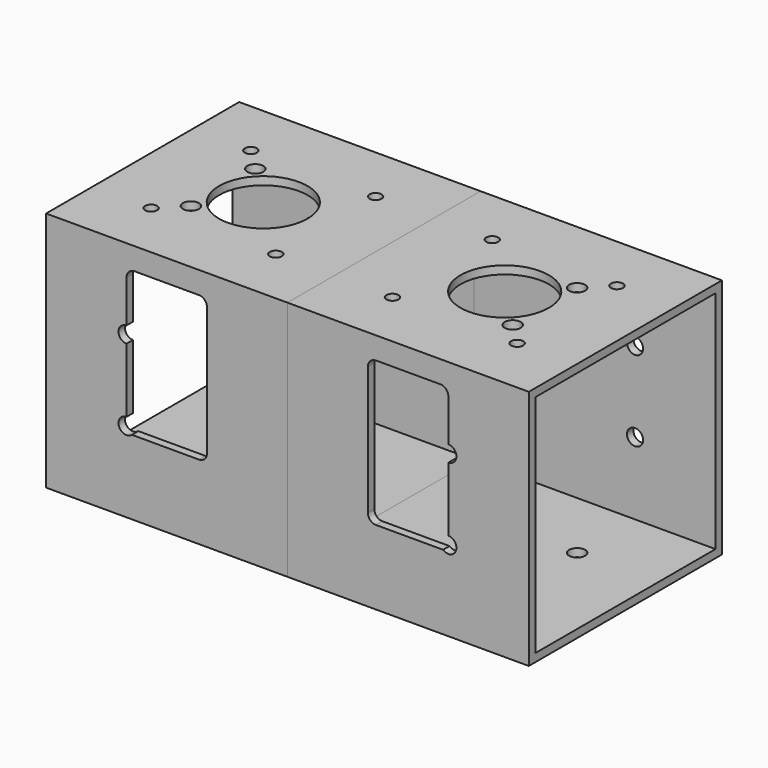
from build123d import *

# Parameters (mm, degrees)
F0_W     = 60
F0_H     = 60
F1_DEPTH = 60
F2_T     = -2
F4_D     = 4
F5_D     = 22
F5_DEPTH = 2
F5_TIP   = 6.6094668093
F6_D     = 3
F6_DEPTH = 2
F6_TIP   = 0.9012909285
F8_D     = 4
F7_W     = 20
F7_H     = 36
F9_DEPTH = 2
F10_R    = 2


with BuildPart() as f1:
    # F0 (on Right) → F1 (new body)
    with BuildSketch(Plane.YZ):
        Rectangle(F0_W, F0_H)
    extrude(amount=-F1_DEPTH)

    # F2
    f2_openings = [f1.faces().sort_by_distance(p)[0] for p in [
        (-60, 0, 0),
        (0, 0, 0),
    ]]
    offset(amount=F2_T, openings=f2_openings)

    # F4 (through all)
    with Locations(Plane.XY.offset(30)):
        with Locations((-40, 10), (-40, -10)):
            Hole(F4_D / 2)

    # F5
    with Locations(Plane.XY.offset(30)):
        with Locations((-30, 0)):
            Hole(F5_D / 2, depth=F5_DEPTH)
            with Locations((0, 0, -(F5_DEPTH + F5_TIP / 2))):  # 118° drill point
                Cone(0, F5_D / 2, F5_TIP, mode=Mode.SUBTRACT)

    # F6
    with Locations(Plane.XY.offset(30)):
        with Locations((-45.5, 15.5), (-14.5, 15.5), (-14.5, -15.5), (-45.5, -15.5)):
            Hole(F6_D / 2, depth=F6_DEPTH)
            with Locations((0, 0, -(F6_DEPTH + F6_TIP / 2))):  # 118° drill point
                Cone(0, F6_D / 2, F6_TIP, mode=Mode.SUBTRACT)

    # F8 (through all)
    with Locations(Plane.XZ.offset(30)):
        with Locations((-40, 10), (-40, -10)):
            Hole(F8_D / 2)

    # F7 (on face) → F9 (cut)
    with BuildSketch(Plane.XZ.offset(30)):
        with Locations((-30, 6.5)):
            Rectangle(F7_W, F7_H)
    extrude(amount=-F9_DEPTH, mode=Mode.SUBTRACT)

    # F10
    f10_edges = [f1.edges().sort_by_distance(p)[0] for p in [
        (-40, -29, 24.5),
        (-20, -29, 24.5),
        (-20, -29, -11.5),
    ]]
    fillet(f10_edges, radius=F10_R)


with BuildPart() as f11_1:
    # F11: instance of F1
    add(f1.part.mirror(Plane.YZ))


solid = Compound([f1.part, f11_1.part])
